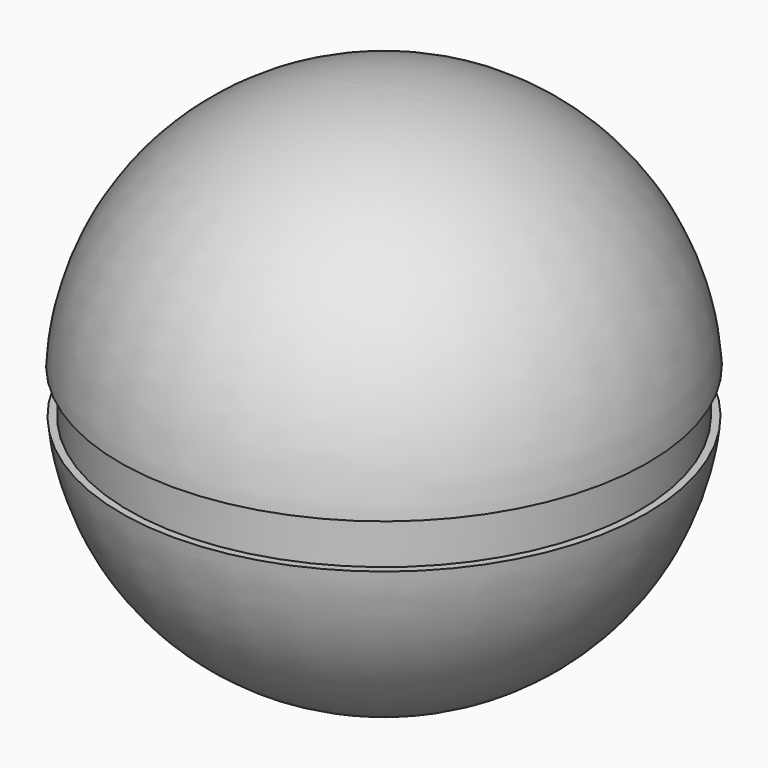
from build123d import *

# Parameters (mm, degrees)
F2_R     = 1.5787292797
F3_DEPTH = 7.8751184046
F4_R     = 1.0079613277
F5_DEPTH = 8.2798842341


with BuildPart() as f1:
    # F0 (on Front) → F1 (revolve)
    with BuildSketch(Plane.XZ):
        with BuildLine():
            Line((0, -7.200146094), (0, 7.5231958181))
            ThreePointArc((0, 7.5231958181), (-5.1783886849, 5.6081211525), (-7.5707412208, 0.6321921246))
            Line((-7.5707412208, 0.6321921246), (-7.5408222763, 0.6321921246))
            Line((-7.5408222763, 0.6321921246), (-7.3254853487, 0.6321921246))
            Line((-7.3254853487, 0.6321921246), (-7.3254853487, -0.6511476797))
            Line((-7.3254853487, -0.6511476797), (-7.5408222763, -0.6511476797))
            ThreePointArc((-7.5408222763, -0.6511476797), (-5.0500980935, -5.399138143), (0, -7.200146094))
        make_face()
    revolve(axis=Axis((0, 0, -2.5440603495), (0, 0, -1)))

    # F4 (on Front) → F5 (join)
    with BuildSketch(Plane.XZ):
        Circle(F4_R)
    extrude(amount=-F5_DEPTH)


with BuildPart() as f3:
    # F2 (on Front) → F3 (new body)
    with BuildSketch(Plane.XZ):
        Circle(F2_R)
    extrude(amount=-F3_DEPTH)


solid = Compound([f1.part, f3.part])
